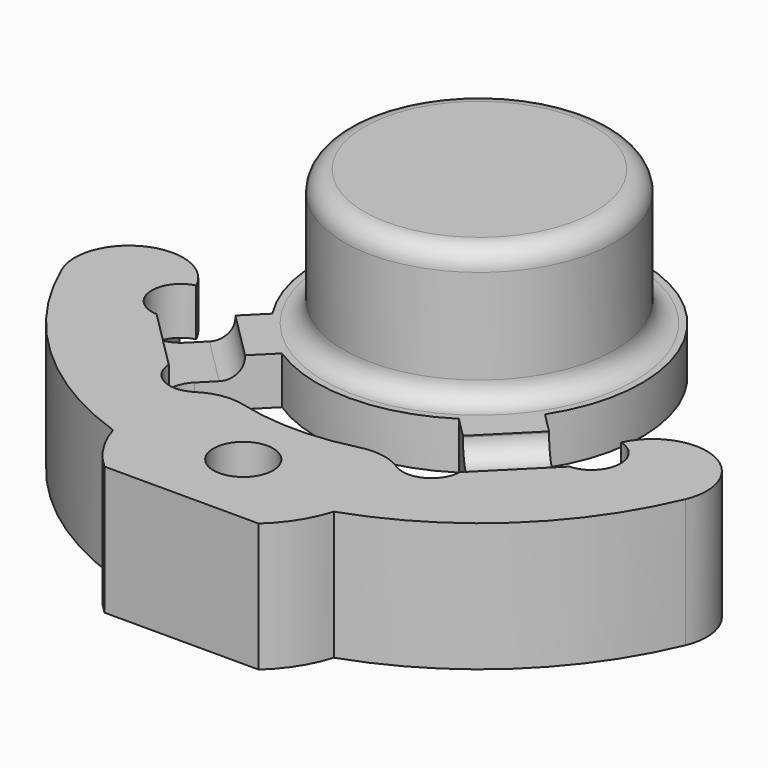
from build123d import *

# Parameters (mm, degrees)
F0_R        = 1.1
F1_DEPTH    = 4.75
F2_R        = 5
F3_DEPTH    = 5
F5_T1_DEPTH = 16.1499020619
F5_T3_DEPTH = 14.3297238483
F5_T5_DEPTH = 10.7226436636
F7_DEPTH    = 0.8
F8_R        = 0.75
F9_R        = 9.625
F10_DEPTH   = 3
F12_R       = 4.5172071506
F12_R_2     = 2.2672071506
F13_DEPTH   = 3.7


# Not quite as in the source:
# - a fillet or chamfer that OpenCascade refuses, or shapes differently, is made with other operations: its cross-section is extruded or revolved along the edge and cut away or added


with BuildPart() as f1:
    # F0 (on Top) → F1 (new body)
    with BuildSketch(Plane.XY):
        with BuildLine():
            Line((-8.3357166343, -1.6650899635), (-12.2050748298, -2.6992866465))
            ThreePointArc((-12.2050748298, -2.6992866465), (-9.3300068577, -8.3187121621), (-4.0757746589, -11.8168549509))
            ThreePointArc((-4.0757746589, -11.8168549509), (-3.593311946, -12.8676823003), (-2.8459674038, -13.75))
            Line((-2.8459674038, -13.75), (2.8459674038, -13.75))
            ThreePointArc((2.8459674038, -13.75), (3.593311946, -12.8676823003), (4.0757746589, -11.8168549509))
            ThreePointArc((4.0757746589, -11.8168549509), (9.3300068577, -8.3187121621), (12.2050748298, -2.6992866465))
            Line((12.2050748298, -2.6992866465), (8.3357166343, -1.6650899635))
            ThreePointArc((8.3357166343, -1.6650899635), (8.1313688943, -2.4774051544), (7.8480653995, -3.2656646917))
            ThreePointArc((7.8480653995, -3.2656646917), (8.5179809488, -4.8326547168), (6.82922604, -5.061459087))
            Line((6.82922604, -5.061459087), (5.0334316447, -3.2656646917))
            ThreePointArc((5.0334316447, -3.2656646917), (0, 6), (-5.0334316447, -3.2656646917))
            Line((-5.0334316447, -3.2656646917), (-6.82922604, -5.061459087))
            ThreePointArc((-6.82922604, -5.061459087), (-8.5179809488, -4.8326547168), (-7.8480653995, -3.2656646917))
            ThreePointArc((-7.8480653995, -3.2656646917), (-8.1313688943, -2.4774051544), (-8.3357166343, -1.6650899635))
        make_face()
        with Locations((0, -10.9)):
            Circle(F0_R, mode=Mode.SUBTRACT)
        with BuildLine():
            Line((-5.061459087, -6.82922604), (-3.2656646917, -5.0334316447))
            ThreePointArc((-3.2656646917, -5.0334316447), (0, -6), (3.2656646917, -5.0334316447))
            Line((3.2656646917, -5.0334316447), (5.061459087, -6.82922604))
            ThreePointArc((5.061459087, -6.82922604), (4.8326547168, -8.5179809488), (3.2656646917, -7.8480653995))
            ThreePointArc((3.2656646917, -7.8480653995), (0, -8.5003938964), (-3.2656646917, -7.8480653995))
            ThreePointArc((-3.2656646917, -7.8480653995), (-4.8326547168, -8.5179809488), (-5.061459087, -6.82922604))
        make_face(mode=Mode.SUBTRACT)
    extrude(amount=F1_DEPTH)

    # F2 (on face) → F3 (join)
    with BuildSketch(Plane.XY.offset(4.75)):
        Circle(F2_R)
    extrude(amount=F3_DEPTH)

    # F5: fillet of radius 2 on 6 edges, made by hand

    # F5_s2 → F5_t1 (cut)
    with BuildSketch(Plane.XY.offset(-5.6999510309)):
        with BuildLine():
            ThreePointArc((10.1863028618, -2.1597120795), (11.4666976063, -3.2135797735), (11.5117544763, -4.871294374))
            ThreePointArc((11.5117544763, -4.871294374), (11.9080394052, -3.801131085), (12.2050748298, -2.6992866465))
            Line((12.2050748298, -2.6992866465), (10.1863028618, -2.1597120795))
        make_face()
        with BuildLine():
            ThreePointArc((-10.1863028618, -2.1597120795), (-11.4666976063, -3.2135797735), (-11.5117544763, -4.871294374))
            ThreePointArc((-11.5117544763, -4.871294374), (-11.9080394052, -3.801131085), (-12.2050748298, -2.6992866465))
            Line((-12.2050748298, -2.6992866465), (-10.1863028618, -2.1597120795))
        make_face()
    extrude(amount=F5_T1_DEPTH, mode=Mode.SUBTRACT)

    # F5_s4 → F5_t3 (cut)
    with BuildSketch(Plane.XY.offset(-4.7898619242)):
        with BuildLine():
            ThreePointArc((10.1866871135, -2.1598147817), (8.7919457915, -2.2951684372), (7.8283732011, -3.3125925525))
            ThreePointArc((7.8283732011, -3.3125925525), (8.1239163121, -2.5017354271), (8.3357166343, -1.6650899635))
            Line((8.3357166343, -1.6650899635), (10.1866871135, -2.1598147817))
        make_face()
        with BuildLine():
            ThreePointArc((-7.8283732011, -3.3125925525), (-8.7919457915, -2.2951684372), (-10.1866871135, -2.1598147817))
            Line((-10.1866871135, -2.1598147817), (-8.3357166343, -1.6650899635))
            ThreePointArc((-8.3357166343, -1.6650899635), (-8.1239163121, -2.5017354271), (-7.8283732011, -3.3125925525))
        make_face()
    extrude(amount=F5_T3_DEPTH, mode=Mode.SUBTRACT)

    # F5_s6 → F5_t5 (cut)
    with BuildSketch(Plane.XY.offset(-2.9863218318)):
        with BuildLine():
            ThreePointArc((3.7221531416, -8.4854887571), (2.954728203, -8.190033245), (2.1332864048, -8.2283525392))
            ThreePointArc((2.1332864048, -8.2283525392), (2.7061638555, -8.0581246938), (3.2656646917, -7.8480653995))
            ThreePointArc((3.2656646917, -7.8480653995), (3.4334814116, -8.2100520192), (3.7221531416, -8.4854887571))
        make_face()
        with BuildLine():
            ThreePointArc((-2.1332864048, -8.2283525392), (-2.954728203, -8.190033245), (-3.7221531416, -8.4854887571))
            ThreePointArc((-3.7221531416, -8.4854887571), (-3.4334814116, -8.2100520192), (-3.2656646917, -7.8480653995))
            ThreePointArc((-3.2656646917, -7.8480653995), (-2.7061638555, -8.0581246938), (-2.1332864048, -8.2283525392))
        make_face()
    extrude(amount=F5_T5_DEPTH, mode=Mode.SUBTRACT)

    # F6 (on face) → F7 (cut)
    with BuildSketch(Plane.XY.offset(4.75)):
        Polygon((4.377220794, -8.6198614811), (8.6198614811, -4.377220794), (7.0098197866, -2.8055128878), (2.7863459937, -7.0289866808), align=None)
        Polygon((-4.377220794, -8.6198614811), (-2.7863459937, -7.0289866808), (-7.0098197866, -2.8055128878), (-8.6198614811, -4.377220794), align=None)
    extrude(amount=-F7_DEPTH, mode=Mode.SUBTRACT)

    # F8
    f8_edges = [f1.edges().sort_by_distance(p)[0] for p in [
        (4.907666, -4.907666, 3.95),
        (-4.907666, -4.907666, 3.95),
        (-5, 0, 4.75),
        (-5, 0, 9.75),
    ]]
    fillet(f8_edges, radius=F8_R)

    # F9 (on Top) → F10 (cut)
    with BuildSketch(Plane.XY):
        Circle(F9_R)
    extrude(amount=F10_DEPTH, mode=Mode.SUBTRACT)

    # F12 (on face) → F13 (cut)
    with BuildSketch(Plane(origin=(0, 0, 3), x_dir=(1, 0, 0), z_dir=(0, 0, -1))):
        Circle(F12_R)
        Circle(F12_R_2, mode=Mode.SUBTRACT)
    extrude(amount=-F13_DEPTH, mode=Mode.SUBTRACT)


solid = f1.part
